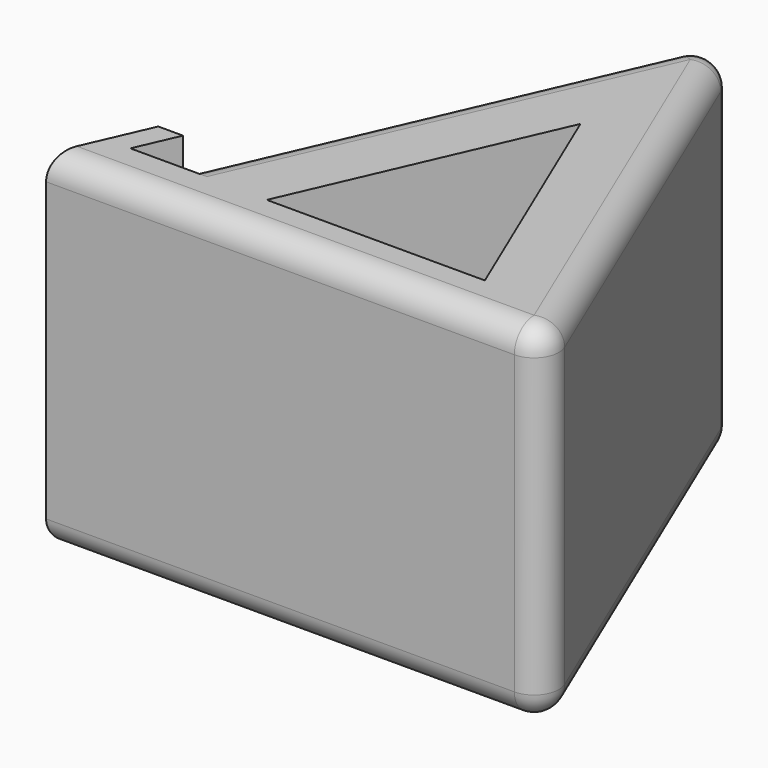
from build123d import *

# Parameters (mm, degrees)
F1_DEPTH     = 70
F2_R         = 5
F3_T1_DEPTH  = 94.0463660375
F3_T6_DEPTH  = 5
F3_T12_DEPTH = 100.881453585
F4_R         = 5
F5_T1_DEPTH  = 107.1682211358
F5_T3_DEPTH  = 60
F5_T8_DEPTH  = 5
F5_T14_DEPTH = 5
F7_DEPTH     = 6
F9_DEPTH     = 70.001


# Not quite as in the source:
# - a fillet or chamfer that OpenCascade refuses, or shapes differently, is made with other operations: its cross-section is extruded or revolved along the edge and cut away or added


with BuildPart() as f1:
    # F0 (on Top) → F1 (new body)
    with BuildSketch(Plane.XY):
        Polygon((8.0247101811, 18.3194985333), (0, 0), (102.2100174067, 0), (59.3825617324, 101.3203288608), (19.2590108271, 9.7228361946), (9.2590108271, 9.7228361946), (13.0247101811, 18.3194985333), align=None)
    extrude(amount=F1_DEPTH)

    # F2
    f2_edges = [f1.edges().sort_by_distance(p)[0] for p in [
        (80.79629, 50.660164, 70),
        (51.105009, 0, 70),
    ]]
    fillet(f2_edges, radius=F2_R)

    # F3: fillet of radius 5 on 2 edges, made by hand

    # F3_s2 → F3_t1 (cut)
    with BuildSketch(Plane.XY.offset(-29.0463660375)):
        with BuildLine():
            ThreePointArc((63.9061324741, 90.6185566458), (59.3330372536, 93.6717493047), (54.7207883471, 90.6780316604))
            Line((54.7207883471, 90.6780316604), (59.3825617324, 101.3203288608))
            Line((59.3825617324, 101.3203288608), (63.9061324741, 90.6185566458))
        make_face()
    extrude(amount=F3_T1_DEPTH, mode=Mode.SUBTRACT)


with BuildPart() as f3_tool4:
    # F3_s5 → F3_t6 (new body)
    with BuildSketch(Plane.XY.offset(65)):
        Polygon((59.3006629805, 88.6718541152), (63.9061324741, 90.6185566458), (59.3825617324, 101.3203288608), (54.7207883471, 90.6780316604), align=None)
    extrude(amount=F3_T6_DEPTH)

    # F3_s7 → F3_t8 (revolve, cut)
    with BuildSketch(Plane(origin=(59.3006629805, 88.6718541152, 65), x_dir=(-0.0064748546, -0.9999790379, 0), z_dir=(-0.9999790379, 0.0064748546, 0))):
        with BuildLine():
            ThreePointArc((0, -5), (5, 0), (0, 5))
            Line((0, 5), (0, -5))
        make_face()
    revolve(axis=Axis((59.3006629805, 88.6718541152, 65), (0, 0, 1)), mode=Mode.SUBTRACT)


with BuildPart() as f1_1:
    add(f1.part)

    # F3_t3: cut F3_tool4
    add(f3_tool4.part, mode=Mode.SUBTRACT)


with BuildPart() as f3_tool10:
    # F3_s11 → F3_t12 (new body)
    with BuildSketch(Plane(origin=(42.135637353, 96.1908566501, 0), x_dir=(0, 0, 1), z_dir=(-0.4012355091, -0.9159749267, 0))):
        with BuildLine():
            ThreePointArc((70, -18.7396238999), (68.5355339059, -15.204089994), (65, -13.7396238999))
            Line((65, -13.7396238999), (70, -13.7396238999))
            Line((70, -13.7396238999), (70, -18.7396238999))
        make_face()
    extrude(amount=F3_T12_DEPTH)

    split(bisect_by=Plane.XZ.offset(-9.7228361946), keep=Keep.BOTTOM)


with BuildPart() as f1_2:
    add(f1_1.part)

    # F3_t9: cut F3_tool10
    add(f3_tool10.part, mode=Mode.SUBTRACT)

    # F4
    f4_edges = [f1_2.edges().sort_by_distance(p)[0] for p in [
        (83.058075, 45.309278, 0),
        (36.9899, 50.200434, 0),
    ]]
    fillet(f4_edges, radius=F4_R)

    # F5: fillet of radius 5 on 1 edges, made by hand

    # F5_s2 → F5_t1 (cut)
    with BuildSketch(Plane.YZ.offset(-12.5)):
        with BuildLine():
            ThreePointArc((5, 0), (1.4644660941, 1.4644660941), (0, 5))
            Line((0, 5), (0, 0))
            Line((0, 0), (5, 0))
        make_face()
    extrude(amount=F5_T1_DEPTH, mode=Mode.SUBTRACT)

    # F5_s4 → F5_t3 (cut)
    with BuildSketch(Plane.XY.offset(5)):
        with BuildLine():
            ThreePointArc((94.6682211358, 0), (98.8355651733, 2.2371674547), (99.2736906295, 6.9467025307))
            Line((99.2736906295, 6.9467025307), (102.2100174067, 0))
            Line((102.2100174067, 0), (94.6682211358, 0))
        make_face()
    extrude(amount=F5_T3_DEPTH, mode=Mode.SUBTRACT)


with BuildPart() as f5_tool6:
    # F5_s7 → F5_t8 (new body)
    with BuildSketch(Plane.XY.offset(65)):
        Polygon((94.6682211358, 5), (94.6682211358, 0), (102.2100174067, 0), (99.2736906295, 6.9467025307), align=None)
    extrude(amount=F5_T8_DEPTH)

    # F5_s9 → F5_t10 (revolve, cut)
    with BuildSketch(Plane(origin=(94.6682211358, 5, 65), x_dir=(-0.8334688075, 0.5525665091, 0), z_dir=(0.5525665091, 0.8334688075, 0))):
        with BuildLine():
            ThreePointArc((0, -5), (5, 0), (0, 5))
            Line((0, 5), (0, -5))
        make_face()
    revolve(axis=Axis((94.6682211358, 5, 65), (0, 0, 1)), mode=Mode.SUBTRACT)


with BuildPart() as f1_3:
    add(f1_2.part)

    # F5_t5: cut F5_tool6
    add(f5_tool6.part, mode=Mode.SUBTRACT)


with BuildPart() as f5_tool12:
    # F5_s13 → F5_t14 (new body)
    with BuildSketch(Plane.XY.offset(5)):
        Polygon((94.6682211358, 5), (99.2736906295, 6.9467025307), (102.2100174067, 0), (94.6682211358, 0), align=None)
    extrude(amount=-F5_T14_DEPTH)

    # F5_s15 → F5_t16 (revolve, cut)
    with BuildSketch(Plane(origin=(94.6682211358, 5, 5), x_dir=(-0.8334688075, 0.5525665091, 0), z_dir=(-0.5525665091, -0.8334688075, 0))):
        with BuildLine():
            ThreePointArc((0, -5), (5, 0), (0, 5))
            Line((0, 5), (0, -5))
        make_face()
    revolve(axis=Axis((94.6682211358, 5, 5), (0, 0, -1)), mode=Mode.SUBTRACT)


with BuildPart() as f1_4:
    add(f1_3.part)

    # F5_t11: cut F5_tool12
    add(f5_tool12.part, mode=Mode.SUBTRACT)

    # F6 (on face) → F7 (cut)
    with BuildSketch(Plane(origin=(0, 0, 0), x_dir=(-0.4012355091, -0.9159749267, 0), z_dir=(-0.9159749267, 0.4012355091, 0))):
        with BuildLine():
            ThreePointArc((-20, 26.7366848613), (-14.1569538303, 29.1569538303), (-11.7366848613, 35))
            ThreePointArc((-11.7366848613, 35), (-14.1569538303, 40.8430461697), (-20, 43.2633151387))
            Line((-20, 43.2633151387), (-20, 26.7366848613))
        make_face()
        with BuildLine():
            Line((-20, 26.7366848613), (-20, 43.2633151387))
            ThreePointArc((-20, 43.2633151387), (-28.2633151387, 35), (-20, 26.7366848613))
        make_face()
    extrude(amount=-F7_DEPTH, mode=Mode.SUBTRACT)

    # F8 (on face) → F9 (cut, through all)
    with BuildSketch(Plane(origin=(0, 0, 0), x_dir=(1, 0, 0), z_dir=(0, 0, -1))):
        Polygon((81.168283108, -9.4247354642), (37.0782896005, -9.4247354642), (59.5163869294, -60.6483537421), align=None)
    extrude(amount=-F9_DEPTH, mode=Mode.SUBTRACT)


solid = f1_4.part
